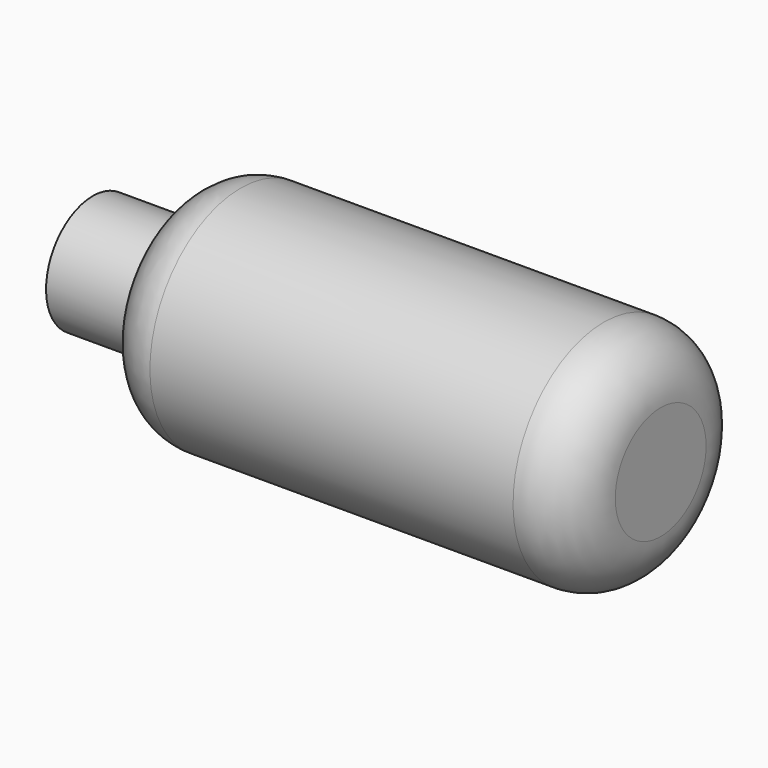
from build123d import *

# Parameters (mm, degrees)
F2_R = 6.35


# Not quite as in the source:
# - a fillet or chamfer that OpenCascade refuses, or shapes differently, is made with other operations: its cross-section is extruded or revolved along the edge and cut away or added


with BuildPart() as f1:
    # F0 (on Front) → F1 (revolve)
    with BuildSketch(Plane.XZ):
        Polygon((-63.5, 0), (0, 0), (0, 12.7), (-53.3020635424, 12.7), (-53.3020635424, 6.5387478179), (-63.5, 6.5387478179), align=None)
    revolve(axis=Axis((-31.75, 0, 0), (-1, 0, 0)))

    # F2
    f2_edges = [f1.edges().sort_by_distance(p)[0] for p in [
        (0, 0, -12.7),
    ]]
    fillet(f2_edges, radius=F2_R)

    # F3: fillet of radius 6.35 on 1 edges, made by hand

    # F3_s1 → F3_t2 (revolve, cut)
    with BuildSketch(Plane.XZ):
        with BuildLine():
            ThreePointArc((-46.9548693385, 12.7), (-51.3777615685, 10.9063718375), (-53.3020635424, 6.5387478179))
            Line((-53.3020635424, 6.5387478179), (-53.3020635424, 12.7))
            Line((-53.3020635424, 12.7), (-46.9548693385, 12.7))
        make_face()
    revolve(axis=Axis((-53.3020635424, 0, 0), (-1, 0, 0)), mode=Mode.SUBTRACT)


solid = f1.part
